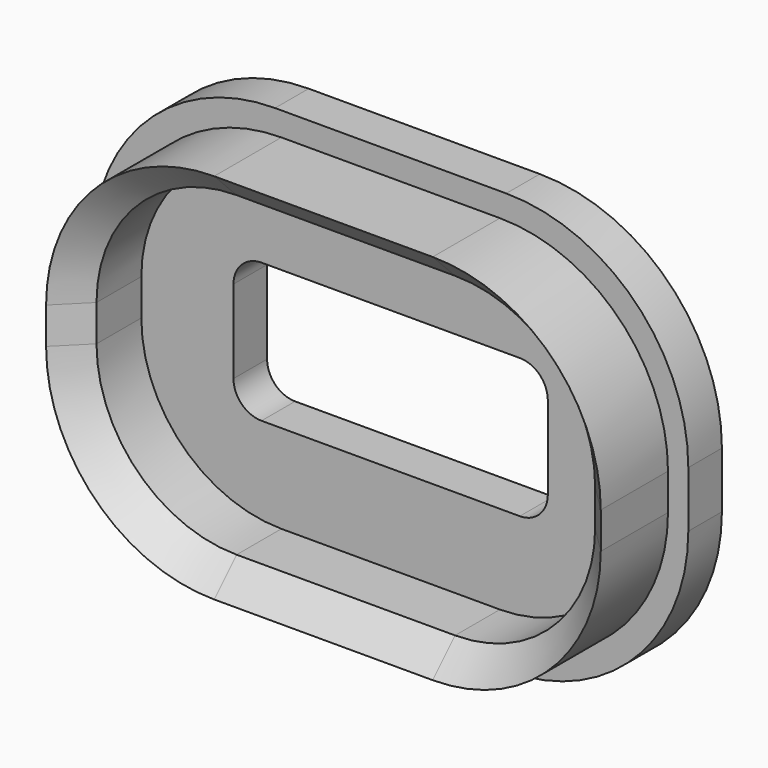
from build123d import *

# Parameters (mm, degrees)
F1_DEPTH = 3.81
F3_DEPTH = 7.62
F5_DEPTH = 3.811
F6_SIZE  = 2.53999


# Not quite as in the source:
# - a fillet or chamfer is up to 0.001 mm smaller than in the source, because OpenCascade refuses the exact size


with BuildPart() as f1:
    # F0 (on Front) → F1 (new body)
    with BuildSketch(Plane.XZ):
        with BuildLine():
            ThreePointArc((-26.9875, -2.54), (-22.1518329574, -14.2143329574), (-10.4775, -19.05))
            Line((-10.4775, -19.05), (10.4775, -19.05))
            ThreePointArc((10.4775, -19.05), (22.1518329574, -14.2143329574), (26.9875, -2.54))
            Line((26.9875, -2.54), (26.9875, 2.54))
            ThreePointArc((26.9875, 2.54), (22.1518329574, 14.2143329574), (10.4775, 19.05))
            Line((10.4775, 19.05), (-10.4775, 19.05))
            ThreePointArc((-10.4775, 19.05), (-22.1518329574, 14.2143329574), (-26.9875, 2.54))
            Line((-26.9875, 2.54), (-26.9875, -2.54))
        make_face()
    extrude(amount=F1_DEPTH)

    # F2 (on face) → F3 (join)
    with BuildSketch(Plane.XZ.offset(3.81)):
        with BuildLine():
            Line((9.906, 16.891), (-9.906, 16.891))
            ThreePointArc((-9.906, 16.891), (-20.6823073453, 12.4273073453), (-25.146, 1.651))
            Line((-25.146, 1.651), (-25.146, -1.651))
            ThreePointArc((-25.146, -1.651), (-20.6823073453, -12.4273073453), (-9.906, -16.891))
            Line((-9.906, -16.891), (9.906, -16.891))
            ThreePointArc((9.906, -16.891), (20.6823073453, -12.4273073453), (25.146, -1.651))
            Line((25.146, -1.651), (25.146, 1.651))
            ThreePointArc((25.146, 1.651), (20.6823073453, 12.4273073453), (9.906, 16.891))
        make_face()
        with BuildLine():
            Line((9.906, -14.351), (-9.906, -14.351))
            ThreePointArc((-9.906, -14.351), (-18.8862561211, -10.6312561211), (-22.606, -1.651))
            Line((-22.606, -1.651), (-22.606, 1.651))
            ThreePointArc((-22.606, 1.651), (-18.8862561211, 10.6312561211), (-9.906, 14.351))
            Line((-9.906, 14.351), (9.906, 14.351))
            ThreePointArc((9.906, 14.351), (18.8862561211, 10.6312561211), (22.606, 1.651))
            Line((22.606, 1.651), (22.606, -1.651))
            ThreePointArc((22.606, -1.651), (18.8862561211, -10.6312561211), (9.906, -14.351))
        make_face(mode=Mode.SUBTRACT)
    extrude(amount=F3_DEPTH)

    # F4 (on face) → F5 (cut, through all)
    with BuildSketch(Plane.XZ.offset(3.81)):
        with BuildLine():
            ThreePointArc((-14.2494, -3.7719), (-13.5054512242, -5.5679512242), (-11.7094, -6.3119))
            Line((-11.7094, -6.3119), (11.7094, -6.3119))
            ThreePointArc((11.7094, -6.3119), (13.5054512242, -5.5679512242), (14.2494, -3.7719))
            Line((14.2494, -3.7719), (14.2494, 3.7719))
            ThreePointArc((14.2494, 3.7719), (13.5054512242, 5.5679512242), (11.7094, 6.3119))
            Line((11.7094, 6.3119), (-11.7094, 6.3119))
            ThreePointArc((-11.7094, 6.3119), (-13.5054512242, 5.5679512242), (-14.2494, 3.7719))
            Line((-14.2494, 3.7719), (-14.2494, -3.7719))
        make_face()
    extrude(amount=-F5_DEPTH, mode=Mode.SUBTRACT)

    # F6 (size 2.54 in the source; OpenCascade refuses exactly that, so slightly less here)
    f6_edges = [f1.edges().sort_by_distance(p)[0] for p in [
        (-18.886256, -11.43, 10.631256),
        (0, -11.43, 14.351),
        (18.886256, -11.43, 10.631256),
        (18.886256, -11.43, -10.631256),
        (-18.886256, -11.43, -10.631256),
        (0, -11.43, -14.351),
        (22.606, -11.43, 0),
        (-22.606, -11.43, 0),
    ]]
    chamfer(f6_edges, length=F6_SIZE)


solid = f1.part
